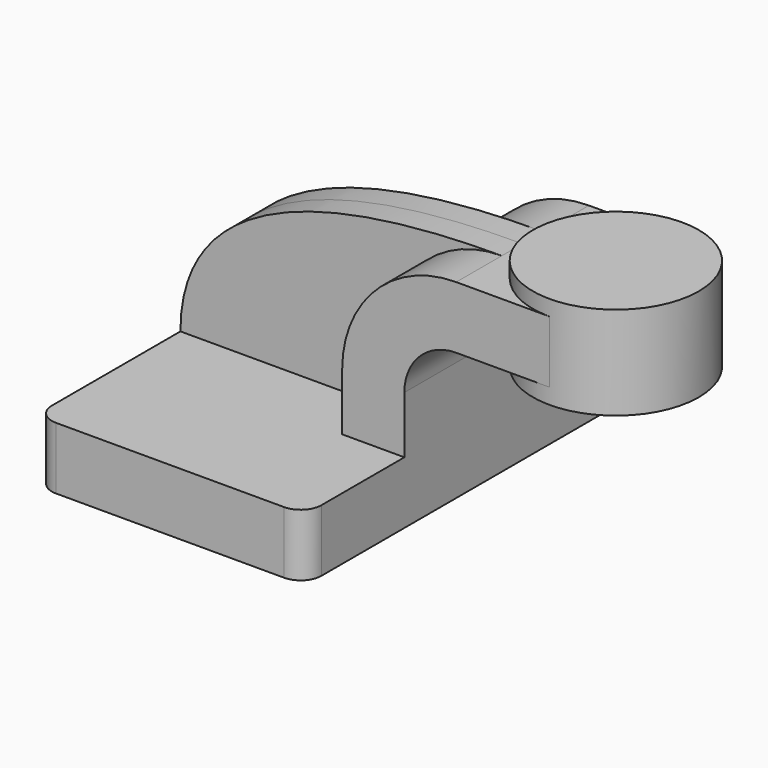
from build123d import *

# Parameters (mm, degrees)
F1_DEPTH = 63.5
F0_W     = 25.4
F0_H     = 19.05
F2_DEPTH = 25.4
F3_DEPTH = 7.9375
F5_R     = 6.35


# Not quite as in the source:
# - a feature names something its author has since deleted; it is built from what else it names


with BuildPart() as f1:
    # F0 (on Front) → F1 (new body, symmetric)
    with BuildSketch(Plane.XZ):
        Polygon((-41.275, 9.525), (-41.275, -9.525), (41.275, -9.525), (41.275, 9.525), (22.225, 9.525), align=None)
    extrude(amount=F1_DEPTH, both=True)

    # F0 (on Front) → F2 (join, symmetric)
    with BuildSketch(Plane.XZ):
        with BuildLine():
            Line((22.225, 9.525), (41.275, 9.525))
            Line((41.275, 9.525), (41.275, 27.0002))
            ThreePointArc((41.275, 27.0002), (45.9246798487, 38.2255201513), (57.15, 42.8752))
            Line((57.15, 42.8752), (60.325, 42.8752))
            Line((60.325, 42.8752), (60.325, 61.9252))
            Line((60.325, 61.9252), (57.15, 61.9252))
            ThreePointArc((57.15, 61.9252), (32.4542956671, 51.6959043329), (22.225, 27.0002))
            Line((22.225, 27.0002), (22.225, 9.525))
        make_face()
        with Locations((73.025, 52.4002)):
            Rectangle(F0_W, F0_H)
    extrude(amount=F2_DEPTH, both=True)

    # F0 (on Front) → F3 (join, symmetric)
    with BuildSketch(Plane.XZ):
        with BuildLine():
            add(Edge.make_bspline(
                [(-41.275, 9.525), (-41.275, 40.5469079711), (-13.9793269336, 61.9252), (57.15, 61.9252)],
                knots=[0, 0, 0, 0, 111.5045361635, 111.5045361635, 111.5045361635, 111.5045361635], degree=3))
            Line((-41.275, 9.525), (22.225, 9.525))
            Line((22.225, 9.525), (22.225, 27.0002))
            ThreePointArc((22.225, 27.0002), (32.4542956671, 51.6959043329), (57.15, 61.9252))
        make_face()
    extrude(amount=F3_DEPTH, both=True)

    # F5
    f5_edges = [f1.edges().sort_by_distance(p)[0] for p in [
        (-41.275, -63.5, 0),
        (41.275, -63.5, 0),
        (41.275, 63.5, 0),
        (-41.275, 63.5, 0),
    ]]
    fillet(f5_edges, radius=F5_R)


with BuildPart() as f4:
    # F0 (on Front) → F4 (revolve)
    with BuildSketch(Plane.XZ):
        Polygon((85.725, 66.675), (85.725, 61.9252), (85.725, 42.8752), (85.725, 38.1), (111.125, 38.1), (111.125, 66.675), align=None)
    revolve(axis=Axis((85.725, 0, 52.3875), (0, 0, 1)))


solid = Compound([f1.part, f4.part])
